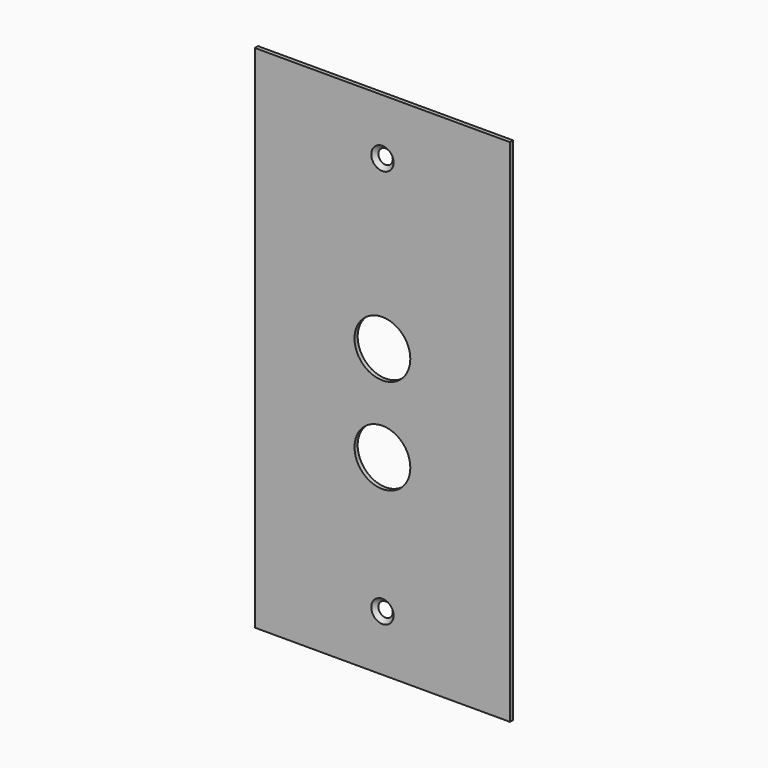
from build123d import *

# Parameters (mm, degrees)
F0_W     = 160
F0_H     = 320
F0_R     = 3
F0_R_2   = 17.5
F1_DEPTH = 2.5


# Not quite as in the source:
# - a fillet or chamfer that OpenCascade refuses, or shapes differently, is made with other operations: its cross-section is extruded or revolved along the edge and cut away or added


with BuildPart() as f1:
    # F0 (on Front) → F1 (new body)
    with BuildSketch(Plane.XZ):
        with Locations((-1.8876045942, 29.6809725389)):
            Rectangle(F0_W, F0_H)
        with Locations((-1.8876045942, -95.3190274611)):
            Circle(F0_R, mode=Mode.SUBTRACT)
        with Locations((-1.8876045942, -10.3190274611)):
            Circle(F0_R_2, mode=Mode.SUBTRACT)
        with Locations((-1.8876045942, 49.6809725389)):
            Circle(F0_R_2, mode=Mode.SUBTRACT)
        with Locations((-1.8876045942, 154.6809725389)):
            Circle(F0_R, mode=Mode.SUBTRACT)
    extrude(amount=F1_DEPTH)

    # F2: chamfer of 4 on 2 edges, made by hand

    # F2_s1 → F2_t2 (revolve, cut)
    with BuildSketch(Plane.XY.offset(154.6809725389)):
        Polygon((1.1123954058, 1.5), (5.1123954058, -2.5), (1.1123954058, -2.5), align=None)
    revolve(axis=Axis((-1.8876045942, -2.5, 154.6809725389), (0, -1, 0)), mode=Mode.SUBTRACT)

    # F2_s3 → F2_t4 (revolve, cut)
    with BuildSketch(Plane.XY.offset(-95.3190274611)):
        Polygon((1.1123954058, 1.5), (5.1123954058, -2.5), (1.1123954058, -2.5), align=None)
    revolve(axis=Axis((-1.8876045942, -2.5, -95.3190274611), (0, -1, 0)), mode=Mode.SUBTRACT)


solid = f1.part
